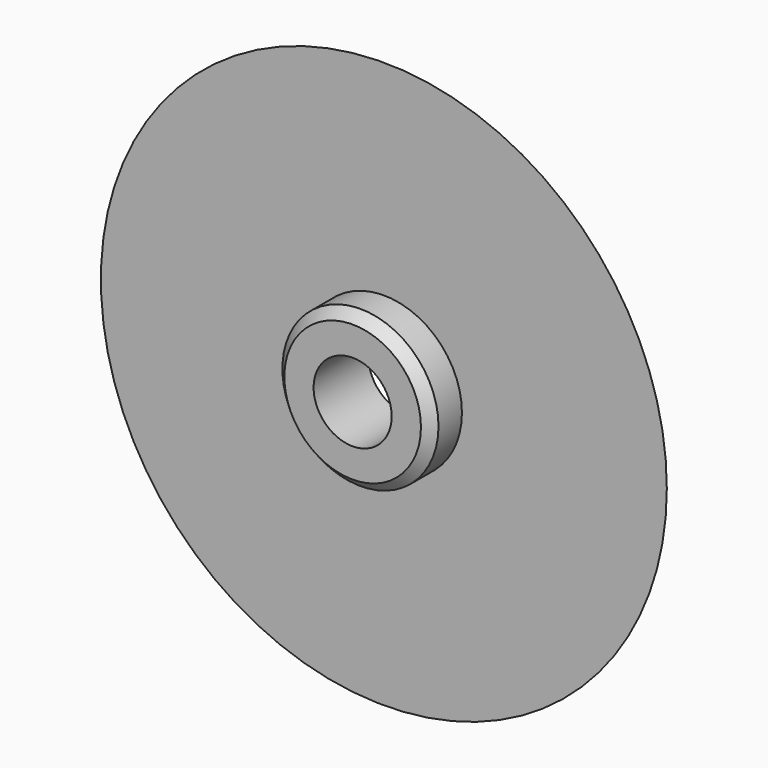
from build123d import *

# Parameters (mm, degrees)
F0_R     = 14.5
F0_R_2   = 4
F1_DEPTH = 1.5
F0_R_3   = 2
F2_DEPTH = 3.5
F3_SIZE  = 0.5


# Not quite as in the source:
# - a fillet or chamfer that OpenCascade refuses, or shapes differently, is made with other operations: its cross-section is extruded or revolved along the edge and cut away or added


with BuildPart() as f1:
    # F0 (on Front) → F1 (new body)
    with BuildSketch(Plane.XZ):
        Circle(F0_R)
        Circle(F0_R_2, mode=Mode.SUBTRACT)
    extrude(amount=F1_DEPTH)

    # F0 (on Front) → F2 (join)
    with BuildSketch(Plane.XZ):
        Circle(F0_R_2)
        Circle(F0_R_3, mode=Mode.SUBTRACT)
    extrude(amount=F2_DEPTH)

    # F3
    f3_edges = [f1.edges().sort_by_distance(p)[0] for p in [
        (-4, -3.5, 0),
    ]]
    chamfer(f3_edges, length=F3_SIZE)

    # F4: fillet of radius 5.08 on 1 edges, made by hand

    # F4_s1 → F4_t2 (revolve, cut)
    with BuildSketch(Plane.XY):
        with BuildLine():
            ThreePointArc((14.5, -1.5), (12.8477578714, -0.3899680172), (10.8958357418, 0))
            Line((10.8958357418, 0), (14.5, 0))
            Line((14.5, 0), (14.5, -1.5))
        make_face()
    revolve(axis=Axis((0, 0, 0), (0, -1, 0)), mode=Mode.SUBTRACT)


solid = f1.part
